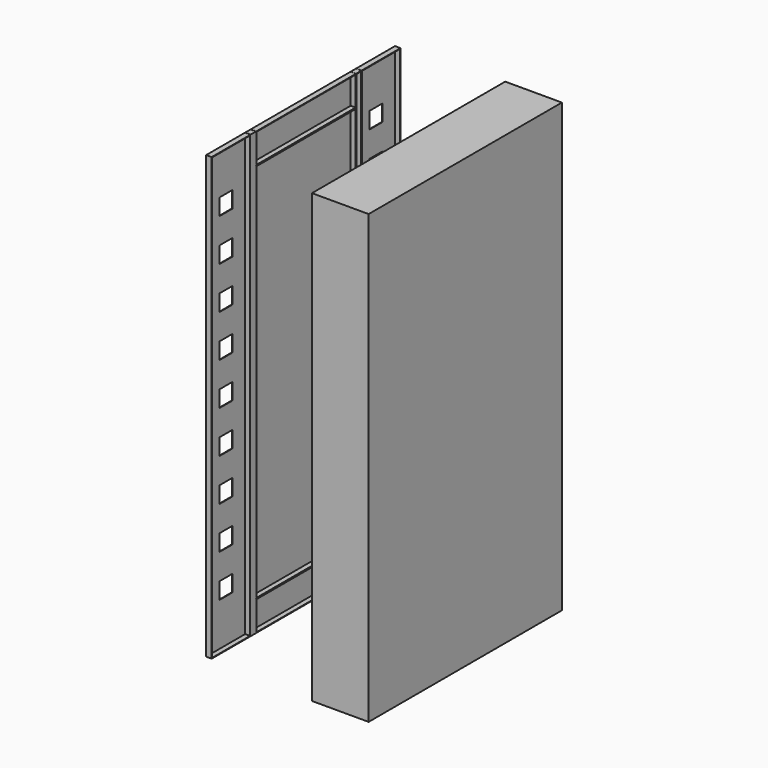
from build123d import *

# Parameters (mm, degrees)
F0_W      = 1100
F0_H      = 2036
F1_DEPTH  = 258
F2_T      = -2.5
F3_W      = 5
F3_H      = 147.5
F3_H_2    = 5
F3_H_3    = 1731
F3_W_2    = 595
F4_DEPTH  = 258
F5_W      = 1100
F5_H      = 2036
F5_W_2    = 1050
F5_H_2    = 1986
F6_DEPTH  = 2.5
F7_R      = 31.5
F8_DEPTH  = 706
F11_DEPTH = 25
F10_W     = 568.4999754384
F10_H     = 137
F10_H_2   = 1734.9996622717
F10_W_2   = 221.0000246707
F10_H_3   = 2010.9996622717
F10_W_3   = 221.5
F12_T     = -2.5
F15_T     = -2.5
F15_2_T   = -2.5
F15_3_T   = -2.5
F15_4_T   = -2.5
F15_5_T   = -2.5
F13_W     = 75
F13_H     = 75
F16_DEPTH = 25
F14_W     = 75
F14_H     = 75
F17_DEPTH = 25


# Not quite as in the source:
# - a feature names something its author has since deleted; it is built from what else it names


with BuildPart() as f1:
    # F0 (on Right) → F1 (new body)
    with BuildSketch(Plane.YZ):
        Rectangle(F0_W, F0_H)
    extrude(amount=-F1_DEPTH)

    # F2
    f2_openings = [f1.faces().sort_by_distance(p)[0] for p in [
        (-258, 0, 0),
    ]]
    offset(amount=F2_T, openings=f2_openings)

    # F3 (on face) → F4 (join)
    with BuildSketch(Plane.YZ):
        with Locations((-300, 944.25)):
            Rectangle(F3_W, F3_H)
        with Locations((-300, 868)):
            Rectangle(F3_W, F3_H_2)
        with Locations((-300, 0)):
            Rectangle(F3_W, F3_H_3)
        with Locations((0, 868)):
            Rectangle(F3_W_2, F3_H_2)
        with Locations((-300, -868)):
            Rectangle(F3_W, F3_H_2)
        with Locations((300, 868)):
            Rectangle(F3_W, F3_H_2)
        with Locations((300, 944.25)):
            Rectangle(F3_W, F3_H)
        with Locations((-300, -944.25)):
            Rectangle(F3_W, F3_H)
        with Locations((0, -868)):
            Rectangle(F3_W_2, F3_H_2)
        with Locations((300, 0)):
            Rectangle(F3_W, F3_H_3)
        with Locations((300, -868)):
            Rectangle(F3_W, F3_H_2)
        with Locations((300, -944.25)):
            Rectangle(F3_W, F3_H)
    extrude(amount=-F4_DEPTH)

    # F5 (on face) → F6 (join)
    with BuildSketch(Plane(origin=(-258, 0, 0), x_dir=(0, -1, 0), z_dir=(-1, 0, 0))):
        Rectangle(F5_W, F5_H)
        Rectangle(F5_W_2, F5_H_2, mode=Mode.SUBTRACT)
    extrude(amount=-F6_DEPTH)

    # F7 (on face) → F8 (cut)
    with BuildSketch(Plane(origin=(0, 302.5, 0), x_dir=(-1, 0, 0), z_dir=(0, 1, 0))):
        with Locations((128.5139412599, 769.34)):
            Circle(F7_R)
        with Locations((130.25, 577.00667)):
            Circle(F7_R)
        with Locations((130.25, 384.67367)):
            Circle(F7_R)
        with Locations((130.25, 192.34067)):
            Circle(F7_R)
        with Locations((130.25, 0.00767)):
            Circle(F7_R)
        with Locations((130.25, -192.32533)):
            Circle(F7_R)
        with Locations((130.25, -384.65833)):
            Circle(F7_R)
        with Locations((130.25, -576.99133)):
            Circle(F7_R)
        with Locations((130.25, -769.32433)):
            Circle(F7_R)
    extrude(amount=-F8_DEPTH, mode=Mode.SUBTRACT)


with BuildPart() as f11:
    # F10 (on offset) → F11 (new body)
    with BuildSketch(Plane.YZ.offset(-750)):
        Polygon((315.4999577856, 1005.5000002704), (285.4999754384, 1005.5000000087), (285.4999754384, -1005.499662263), (315.4999753293, -1005.4996620013), align=None)
    extrude(amount=F11_DEPTH)

    # F12
    f12_openings = [f11.faces().sort_by_distance(p)[0] for p in [
        (-725, 300.499971, 7.1e-05),
    ]]
    offset(amount=F12_T, openings=f12_openings)


with BuildPart() as f11b:
    # F10 (on offset) → F11, piece 2 (new body)
    with BuildSketch(Plane.YZ.offset(-750)):
        Polygon((-285, 1005.5), (-300, 1005.5), (-315, 1005.5), (-315, -1005.4996622717), (-285, -1005.4996622717), align=None)
    extrude(amount=F11_DEPTH)


with BuildPart() as f11c:
    # F10 (on offset) → F11, piece 3 (new body)
    with BuildSketch(Plane.YZ.offset(-750)):
        with Locations((0.2499877192, 937)):
            Rectangle(F10_W, F10_H)
    extrude(amount=F11_DEPTH)

    # F15#4
    f15_4_openings = [f11c.faces().sort_by_distance(p)[0] for p in [
        (-725, 0.249988, 937),
    ]]
    offset(amount=F15_4_T, openings=f15_4_openings)


with BuildPart() as f11d:
    # F10 (on offset) → F11, piece 4 (new body)
    with BuildSketch(Plane.YZ.offset(-750)):
        with Locations((0.2499877192, -936.9996622717)):
            Rectangle(F10_W, F10_H)
    extrude(amount=F11_DEPTH)

    # F15#5
    f15_5_openings = [f11d.faces().sort_by_distance(p)[0] for p in [
        (-725, 0.249988, -936.999662),
    ]]
    offset(amount=F15_5_T, openings=f15_5_openings)


with BuildPart() as f11e:
    # F10 (on offset) → F11, piece 5 (new body)
    with BuildSketch(Plane.YZ.offset(-750)):
        with Locations((0.2499877192, 0.0001688641)):
            Rectangle(F10_W, F10_H_2)
    extrude(amount=F11_DEPTH)

    # F15#3
    f15_3_openings = [f11e.faces().sort_by_distance(p)[0] for p in [
        (-725, 0.249988, 0.000169),
    ]]
    offset(amount=F15_3_T, openings=f15_3_openings)


with BuildPart() as f11f:
    # F10 (on offset) → F11, piece 6 (new body)
    with BuildSketch(Plane.YZ.offset(-750)):
        with Locations((426.9999876647, 0.0001691346)):
            Rectangle(F10_W_2, F10_H_3)
    extrude(amount=F11_DEPTH)

    # F15
    f15_openings = [f11f.faces().sort_by_distance(p)[0] for p in [
        (-725, 426.999988, 0.000169),
    ]]
    offset(amount=F15_T, openings=f15_openings)

    # F13 (on face) → F16 (cut)
    with BuildSketch(Plane(origin=(-750, 0, 0), x_dir=(0, -1, 0), z_dir=(-1, 0, 0))):
        with Locations((-426.9999876647, -769.32433)):
            Rectangle(F13_W, F13_H)
        with Locations((-426.9999876647, -576.99133)):
            Rectangle(F13_W, F13_H)
        with Locations((-426.9999876647, -384.65833)):
            Rectangle(F13_W, F13_H)
        with Locations((-426.9999876647, -192.32533)):
            Rectangle(F13_W, F13_H)
        with Locations((-426.9999876647, 0.00767)):
            Rectangle(F13_W, F13_H)
        with Locations((-426.9999876647, 192.34067)):
            Rectangle(F13_W, F13_H)
        with Locations((-426.9999876647, 384.67367)):
            Rectangle(F13_W, F13_H)
        with Locations((-426.9999876647, 577.00667)):
            Rectangle(F13_W, F13_H)
        with Locations((-426.9999876647, 769.34)):
            Rectangle(F13_W, F13_H)
    extrude(amount=-F16_DEPTH, mode=Mode.SUBTRACT)


with BuildPart() as f11g:
    # F10 (on offset) → F11, piece 7 (new body)
    with BuildSketch(Plane.YZ.offset(-750)):
        with Locations((-426.75, 0.0001688641)):
            Rectangle(F10_W_3, F10_H_3)
    extrude(amount=F11_DEPTH)

    # F15#2
    f15_2_openings = [f11g.faces().sort_by_distance(p)[0] for p in [
        (-725, -426.75, 0.000169),
    ]]
    offset(amount=F15_2_T, openings=f15_2_openings)

    # F14 (on face) → F17 (cut)
    with BuildSketch(Plane(origin=(-750, 0, 0), x_dir=(0, -1, 0), z_dir=(-1, 0, 0))):
        with Locations((426.75, -769.32433)):
            Rectangle(F14_W, F14_H)
        with Locations((426.75, -576.99133)):
            Rectangle(F14_W, F14_H)
        with Locations((426.75, -384.65833)):
            Rectangle(F14_W, F14_H)
        with Locations((426.75, -192.32533)):
            Rectangle(F14_W, F14_H)
        with Locations((426.75, 0.00767)):
            Rectangle(F14_W, F14_H)
        with Locations((426.75, 192.34067)):
            Rectangle(F14_W, F14_H)
        with Locations((426.75, 577.00667)):
            Rectangle(F14_W, F14_H)
        with Locations((426.75, 769.34)):
            Rectangle(F14_W, F14_H)
        with Locations((426.75, 384.67367)):
            Rectangle(F14_W, F14_H)
    extrude(amount=-F17_DEPTH, mode=Mode.SUBTRACT)


solid = Compound([f1.part, f11.part, f11b.part, f11c.part, f11d.part, f11e.part, f11f.part, f11g.part])
